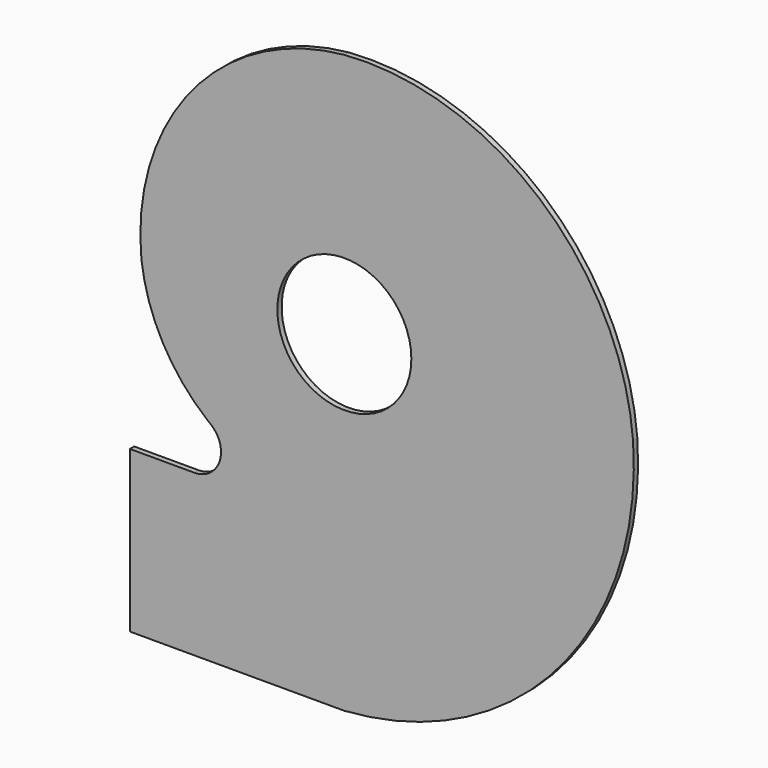
from build123d import *

# Parameters (mm, degrees)
F0_R     = 125
F1_DEPTH = 10


# Not quite as in the source:
# - a feature names something its author has since deleted; it is built from what else it names


with BuildPart() as f1:
    # F0 (on Front) → F1 (new body)
    with BuildSketch(Plane.XZ):
        with BuildLine():
            ThreePointArc((0, -618.6190456596), (397.429722157, -420.8611796621), (538.6190456596, 0))
            ThreePointArc((538.6190456596, 0), (364.2926371672, 340.8611796621), (0, 458.6190456596))
            ThreePointArc((0, 458.6190456596), (-284.2926371672, 307.7240946723), (-378.6190456596, 0))
            ThreePointArc((-378.6190456596, 0), (-338.9932719851, -123.9081492515), (-255.845498181, -223.9575325662))
            Line((-255.845498181, -223.9575325662), (-248.8807463186, -229.5026751274))
            ThreePointArc((-248.8807463186, -229.5026751274), (-232.823383589, -285.1142187928), (-280.0241173048, -318.6190456596))
            Line((-280.0241173048, -318.6190456596), (-400, -318.6190456596))
            Line((-400, -318.6190456596), (-400, -618.6190456596))
            Line((-400, -618.6190456596), (0, -618.6190456596))
        make_face()
        Circle(F0_R, mode=Mode.SUBTRACT)
    extrude(amount=F1_DEPTH)


solid = f1.part
